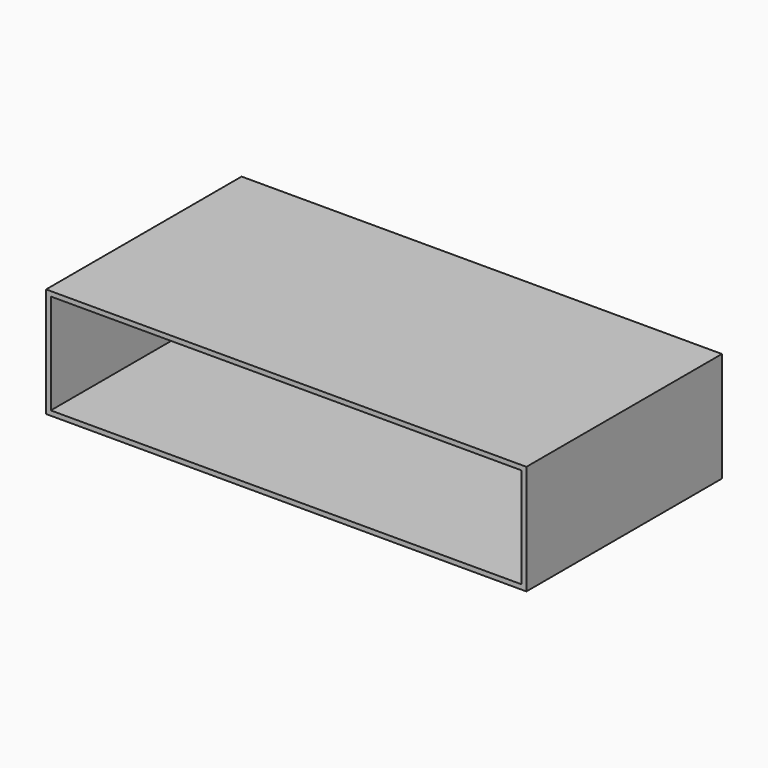
from build123d import *

# Parameters (mm, degrees)
F0_W     = 1020
F0_H     = 233
F0_W_2   = 1000
F0_H_2   = 213
F1_DEPTH = 509
F2_W     = 1020
F2_H     = 233
F2_W_2   = 1000
F2_H_2   = 213
F3_DEPTH = 10


with BuildPart() as f1:
    # F0 (on Front) → F1 (new body)
    with BuildSketch(Plane.XZ):
        with Locations((0, 106.5)):
            Rectangle(F0_W, F0_H)
        with Locations((0, 106.5)):
            Rectangle(F0_W_2, F0_H_2, mode=Mode.SUBTRACT)
    extrude(amount=-F1_DEPTH)

    # F2 (on face) → F3 (join)
    with BuildSketch(Plane(origin=(0, 509, 0), x_dir=(-1, 0, 0), z_dir=(0, 1, 0))):
        with Locations((0, 106.5)):
            Rectangle(F2_W, F2_H)
        with Locations((0, 106.5)):
            Rectangle(F2_W_2, F2_H_2, mode=Mode.SUBTRACT)
        with Locations((0, 106.5)):
            Rectangle(F2_W_2, F2_H_2)
    extrude(amount=F3_DEPTH)


solid = f1.part
